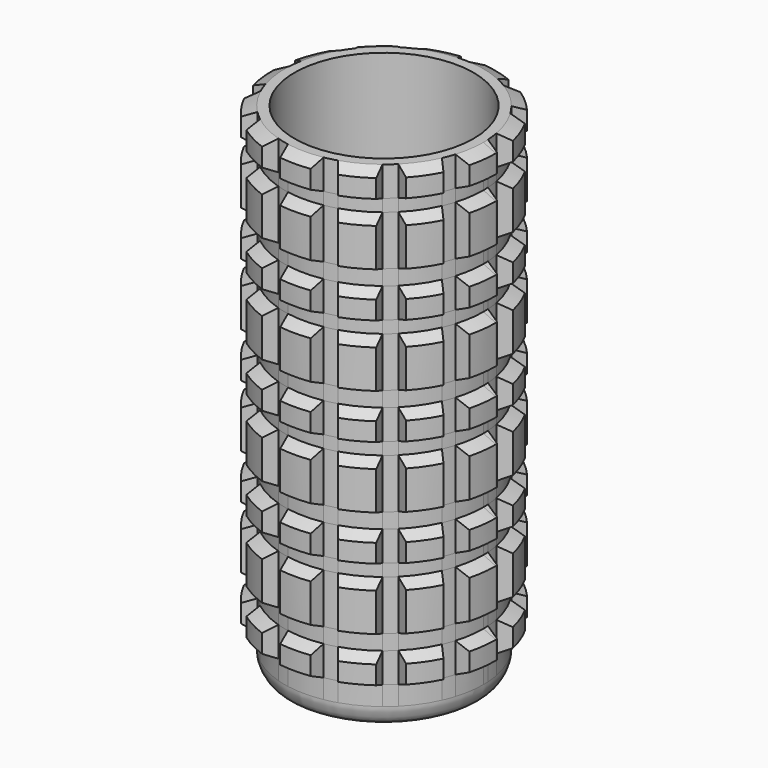
from build123d import *
from build123d import SkipClean  # not in build123d's __all__

# Parameters (mm, degrees)
F6_DEPTH = 264.5481982434


# Not quite as in the source:
# - a feature names something its author has since deleted; it is built from what else it names


with BuildPart() as f1:
    # F0 (on Front) → F1 (revolve)
    with BuildSketch(Plane.XZ):
        with BuildLine():
            Line((50, -115), (50, 125))
            Line((50, 125), (45, 125))
            Line((45, 125), (45, -115))
            ThreePointArc((45, -115), (44.6057132656, -117.3997581102), (43.4643096033, -119.5471981434))
            ThreePointArc((43.4643096033, -119.5471981435), (21.8507621163, -116.1398932421), (0, -115))
            Line((0, -115), (0, -120))
            ThreePointArc((0, -120), (21.3305058754, -121.1127529268), (42.429445089, -124.438931521))
            ThreePointArc((42.429445089, -124.438931521), (45.2044309311, -124.2346257711), (47.4405160055, -122.5786635724))
            ThreePointArc((47.4405160055, -122.5786635724), (49.3428554426, -118.9995968504), (50, -115))
        make_face()
    revolve(axis=Axis((0, 0, 2.5), (0, 0, 1)))

    # F2 (on Front) → F3 (revolve)
    with BuildSketch(Plane.XZ):
        Polygon((56.1803398875, 122.1180601805), (50, 125), (50, 110), (56.1803398875, 112.8819398195), align=None)
        Polygon((56.1803398875, 100.937720293), (50, 103.8196601125), (50, 78.8196601125), (56.1803398875, 81.7015999321), align=None)
        Polygon((56.1803398875, 68.2984000679), (50, 71.1803398875), (50, 56.1803398875), (56.1803398875, 59.062279707), align=None)
        Polygon((56.1803398875, 47.1180601805), (50, 50), (50, 25), (56.1803398875, 27.8819398195), align=None)
        Polygon((56.1803398875, 14.4787399554), (50, 17.3606797749), (50, 2.3606797749), (56.1803398875, 5.2426195945), align=None)
        Polygon((56.1803398875, -6.7015999321), (50, -3.8196601125), (50, -28.8196601125), (56.1803398875, -25.937720293), align=None)
        Polygon((56.1803398875, -39.3409201571), (50, -36.4589803376), (50, -51.4589803376), (56.1803398875, -48.5770405181), align=None)
        Polygon((56.1803398875, -60.5212600446), (50, -57.6393202251), (50, -82.6393202251), (56.1803398875, -79.7573804055), align=None)
        Polygon((56.1803398875, -93.1605802697), (50, -90.2786404501), (50, -105.2786404501), (56.1803398875, -102.3967006306), align=None)
    revolve(axis=Axis((0, 0, 2.5), (0, 0, 1)))

    # F5 (on offset) → F6 (cut, through all)
    with BuildSketch(Plane.XY.offset(140)):
        with BuildLine():
            ThreePointArc((-21.0204474313, 57.6375741779), (-28.569647411, 54.4349151766), (-35.4938184714, 50.0413630675))
            Line((-35.4938184714, 50.0413630675), (-25.9279486276, 42.7520932817))
            ThreePointArc((-25.9279486276, 42.7520932817), (-23.2361586022, 44.2728012827), (-20.4555294336, 45.6242404385))
            Line((-20.4555294336, 45.6242404385), (-21.0204474313, 57.6375741779))
        make_face()
        with BuildLine():
            ThreePointArc((-3.0901699437, 49.9044171364), (0, 50), (3.0901699437, 49.9044171364))
            Line((3.0901699437, 49.9044171364), (8.1728344609, 60.804226368))
            ThreePointArc((8.1728344609, 60.804226368), (0, 61.4767008181), (-8.1728344609, 60.804226368))
            Line((-8.1728344609, 60.804226368), (-3.0901699437, 49.9044171364))
        make_face()
        with BuildLine():
            ThreePointArc((35.4938184714, 50.0413630675), (28.569647411, 54.4349151766), (21.0204474313, 57.6375741779))
            Line((21.0204474313, 57.6375741779), (20.4555294336, 45.6242404385))
            ThreePointArc((20.4555294336, 45.6242404385), (23.2361586022, 44.2728012827), (25.9279486276, 42.7520932817))
            Line((25.9279486276, 42.7520932817), (35.4938184714, 50.0413630675))
        make_face()
        with BuildLine():
            ThreePointArc((-45.3981981409, 41.2668483518), (-50.5943329016, 34.9227464801), (-54.6835964171, 27.814626552))
            Line((-54.6835964171, 27.814626552), (-42.8259467465, 25.8057800748))
            ThreePointArc((-42.8259467465, 25.8057800748), (-41.1491932947, 28.4032373366), (-39.3151135336, 30.8921000879))
            Line((-39.3151135336, 30.8921000879), (-45.3981981409, 41.2668483518))
        make_face()
        with BuildLine():
            ThreePointArc((-59.375768764, 15.4423848877), (-61.0284664524, 7.4101974297), (-61.3460214323, -0.7841057039))
            Line((-61.3460214323, -0.7841057039), (-49.9130365744, 2.9476736461))
            ThreePointArc((-49.9130365744, 2.9476736461), (-49.6354437049, 6.0268340128), (-49.1680789215, 9.0829518973))
            Line((-49.1680789215, 9.0829518973), (-59.375768764, 15.4423848877))
        make_face()
        with BuildLine():
            ThreePointArc((-59.7510663188, -13.9197428532), (-57.4817138116, -21.7999385493), (-53.9548122372, -29.2032087926))
            Line((-53.9548122372, -29.2032087926), (-45.5656512404, -20.5857092916))
            ThreePointArc((-45.5656512404, -20.5857092916), (-46.7508121343, -17.7302443521), (-47.7572299681, -14.8069911115))
            Line((-47.7572299681, -14.8069911115), (-59.7510663188, -13.9197428532))
        make_face()
        with BuildLine():
            ThreePointArc((-46.4381146584, -40.0930252576), (-40.7665932664, -46.0159713244), (-34.2032057844, -50.9322086837))
            Line((-34.2032057844, -50.9322086837), (-30.7797243329, -39.4031543153))
            ThreePointArc((-30.7797243329, -39.4031543153), (-33.156132912, -37.4255374086), (-35.405775166, -35.3048309003))
            Line((-35.405775166, -35.3048309003), (-46.4381146584, -40.0930252576))
        make_face()
        with BuildLine():
            ThreePointArc((-22.4867505697, -57.0814787488), (-14.7123374945, -59.6902996217), (-6.6160570798, -60.993253365))
            Line((-6.6160570798, -60.993253365), (-8.9425335165, -49.1938115448))
            ThreePointArc((-8.9425335165, -49.1938115448), (-11.9657832144, -48.5470908713), (-14.9432839592, -47.7147593991))
            Line((-14.9432839592, -47.7147593991), (-22.4867505697, -57.0814787488))
        make_face()
        with BuildLine():
            ThreePointArc((6.6160570798, -60.993253365), (14.7123374945, -59.6902996217), (22.4867505697, -57.0814787488))
            Line((22.4867505697, -57.0814787488), (14.9432839592, -47.7147593991))
            ThreePointArc((14.9432839592, -47.7147593991), (11.9657832144, -48.5470908713), (8.9425335165, -49.1938115448))
            Line((8.9425335165, -49.1938115448), (6.6160570798, -60.993253365))
        make_face()
        with BuildLine():
            ThreePointArc((34.2032057844, -50.9322086837), (40.7665932664, -46.0159713244), (46.4381146584, -40.0930252576))
            Line((46.4381146584, -40.0930252576), (35.405775166, -35.3048309003))
            ThreePointArc((35.405775166, -35.3048309003), (33.156132912, -37.4255374086), (30.7797243329, -39.4031543153))
            Line((30.7797243329, -39.4031543153), (34.2032057844, -50.9322086837))
        make_face()
        with BuildLine():
            ThreePointArc((53.9548122372, -29.2032087926), (57.4817138116, -21.7999385493), (59.7510663188, -13.9197428532))
            Line((59.7510663188, -13.9197428532), (47.7572299681, -14.8069911115))
            ThreePointArc((47.7572299681, -14.8069911115), (46.7508121343, -17.7302443521), (45.5656512404, -20.5857092916))
            Line((45.5656512404, -20.5857092916), (53.9548122372, -29.2032087926))
        make_face()
        with BuildLine():
            ThreePointArc((61.3460214323, -0.7841057039), (61.0284664524, 7.4101974297), (59.375768764, 15.4423848877))
            Line((59.375768764, 15.4423848877), (49.1680789215, 9.0829518973))
            ThreePointArc((49.1680789215, 9.0829518973), (49.6354437049, 6.0268340128), (49.9130365744, 2.9476736461))
            Line((49.9130365744, 2.9476736461), (61.3460214323, -0.7841057039))
        make_face()
        with BuildLine():
            ThreePointArc((54.6835964171, 27.814626552), (50.5943329016, 34.9227464801), (45.3981981409, 41.2668483518))
            Line((45.3981981409, 41.2668483518), (39.3151135336, 30.8921000879))
            ThreePointArc((39.3151135336, 30.8921000879), (41.1491932947, 28.4032373366), (42.8259467465, 25.8057800748))
            Line((42.8259467465, 25.8057800748), (54.6835964171, 27.814626552))
        make_face()
    with SkipClean():  # cleaning this boolean's faces spoils the solid; the shape is the same uncleaned
        extrude(amount=-F6_DEPTH, mode=Mode.SUBTRACT)


solid = f1.part
